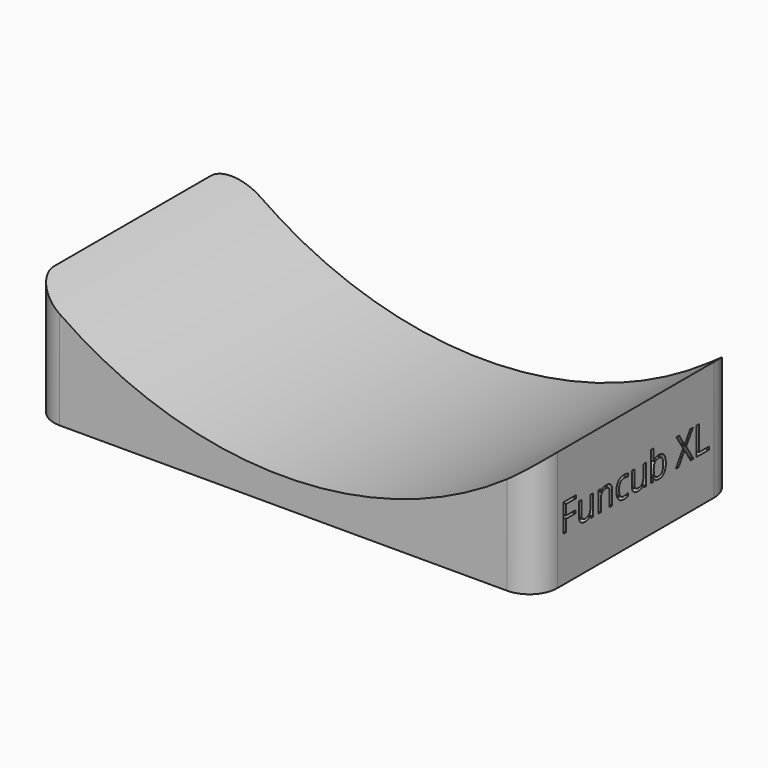
from build123d import *

# Parameters (mm, degrees)
F1_DEPTH     = 40
F3_DEPTH     = 45.001
F4_TEXT_SIZE = 6.9444444444
F5_DEPTH     = 1


# Not quite as in the source:
# - Text() gives the source's letters only with a copy of the font that has no kerning and outlines rounded to 1/6400 em; it was checked with that copy


with BuildPart() as f1:
    # F0 (on Top) → F1 (new body)
    with BuildSketch(Plane.XY):
        with BuildLine():
            Line((40, 22.5), (-40, 22.5))
            ThreePointArc((-40, 22.5), (-43.5355339059, 21.0355339059), (-45, 17.5))
            Line((-45, 17.5), (-45, -17.5))
            ThreePointArc((-45, -17.5), (-43.5355339059, -21.0355339059), (-40, -22.5))
            Line((-40, -22.5), (40, -22.5))
            ThreePointArc((40, -22.5), (43.5355339059, -21.0355339059), (45, -17.5))
            Line((45, -17.5), (45, 17.5))
            ThreePointArc((45, 17.5), (43.5355339059, 21.0355339059), (40, 22.5))
        make_face()
    extrude(amount=F1_DEPTH)

    # F2 (on face) → F3 (cut, through all)
    with BuildSketch(Plane.XZ.offset(22.5)):
        with BuildLine():
            Line((60.6217782649, 40), (-60.6217782649, 40))
            ThreePointArc((-60.6217782649, 40), (0, 5), (60.6217782649, 40))
        make_face()
    extrude(amount=-F3_DEPTH, mode=Mode.SUBTRACT)

    # F4 (on face) → F5 (cut)
    with BuildSketch(Plane.YZ.offset(45)):
        with Locations((-16.8202039931, 8.00189705)):
            Text('Funcub XL', F4_TEXT_SIZE, font='Open Sans', text_align=(TextAlign.LEFT, TextAlign.BOTTOM))
    extrude(amount=-F5_DEPTH, mode=Mode.SUBTRACT)


solid = f1.part
